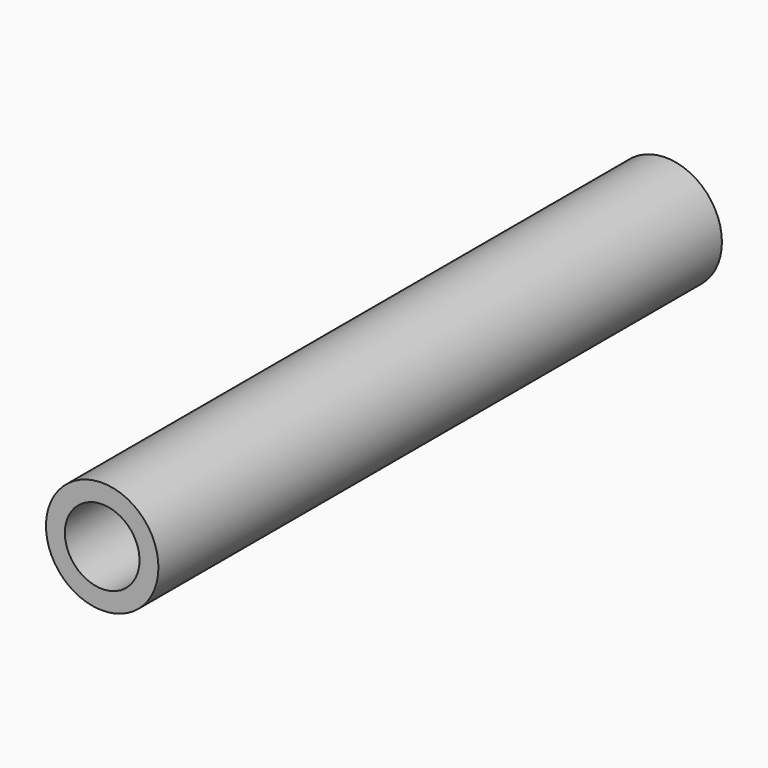
from build123d import *

# Parameters (mm, degrees)
F0_R     = 2.0275396845
F1_DEPTH = 25.4
F2_R     = 1.3462
F3_DEPTH = 25.4


# Not quite as in the source:
# - a feature names something its author has since deleted; it is built from what else it names


with BuildPart() as f1:
    # F0 (on Front) → F1 (new body)
    with BuildSketch(Plane.XZ):
        with Locations((-4.829290323, -1.1499428656)):
            Circle(F0_R)
    extrude(amount=F1_DEPTH)

    # F2 (on face) → F3 (cut)
    with BuildSketch(Plane(origin=(0, 0, 0), x_dir=(-1, 0, 0), z_dir=(0, 1, 0))):
        with Locations((4.829290323, -1.1499428656)):
            Circle(F2_R)
    extrude(amount=-F3_DEPTH, mode=Mode.SUBTRACT)


solid = f1.part
